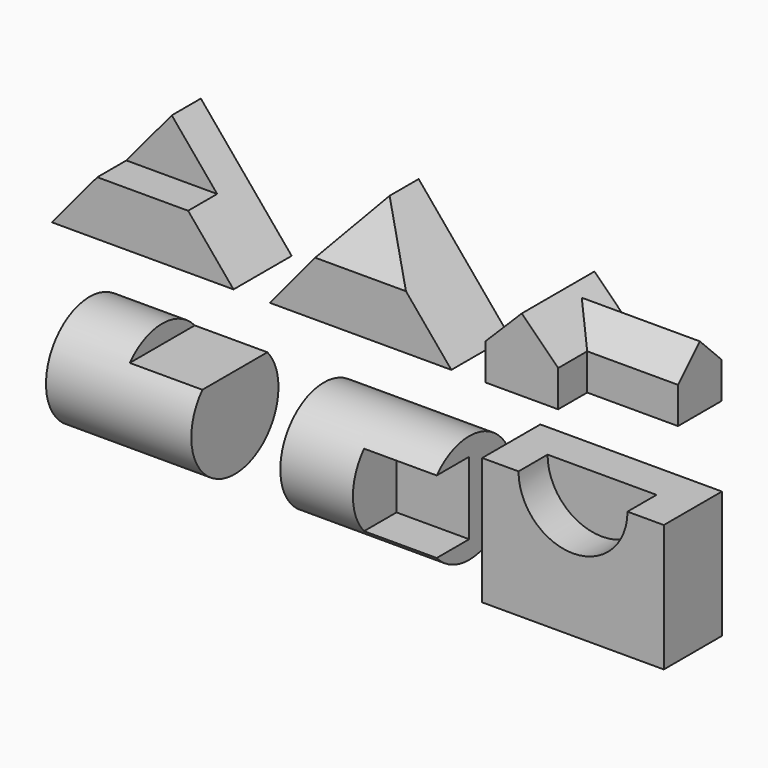
from build123d import *

# Parameters (mm, degrees)
F1_DEPTH  = 101.6
F3_DEPTH  = 50.8
F5_DEPTH  = 101.6
F9_DEPTH  = 63.5
F11_DEPTH = 127
F15_R     = 76.2
F16_DEPTH = 203.2
F18_DEPTH = 101.6
F20_R     = 76.2
F21_DEPTH = 203.2
F23_DEPTH = 101.6
F25_DEPTH = 101.6
F27_DEPTH = 50.8


with BuildPart() as f1:
    # F0 (on Front) → F1 (new body)
    with BuildSketch(Plane.XZ):
        Polygon((127, 152.4), (0, 0), (254, 0), align=None)
    extrude(amount=-F1_DEPTH)

    # F2 (on face) → F3 (cut)
    with BuildSketch(Plane.XZ):
        Polygon((63.5, 76.2), (127, 76.2), (190.5, 76.2), (127, 152.4), align=None)
    extrude(amount=-F3_DEPTH, mode=Mode.SUBTRACT)


with BuildPart() as f5:
    # F4 (on Front) → F5 (new body)
    with BuildSketch(Plane.XZ):
        Polygon((431.6333237171, 152.4), (304.6333237171, 0), (558.6333237171, 0), align=None)
    extrude(amount=-F5_DEPTH)

    # F8 (on 3pt) → F9 (cut, symmetric)
    with BuildSketch(Plane.YZ.offset(431.6333237171)):
        Polygon((50.8, 152.4), (0, 152.4), (0, 76.2), align=None)
    extrude(amount=F9_DEPTH, both=True, mode=Mode.SUBTRACT)


with BuildPart() as f11:
    # F10 (on Front) → F11 (new body)
    with BuildSketch(Plane.XZ):
        Polygon((606.3837154388, 50.8), (606.3837154388, 0), (657.1837154388, 0), (707.9837154388, 0), (707.9837154388, 50.8), (657.1837154388, 101.6), align=None)
    extrude(amount=-F11_DEPTH)

    # F13 (on offset) → F14 (join, up to the next surface of F11)
    with BuildSketch(Plane.YZ.offset(834.9837154388)):
        Polygon((88.9, 88.9), (50.8, 50.8), (50.8, 0), (127, 0), (127, 50.8), align=None)
    extrude(until=Until.NEXT, dir=(-1, 0, 0))


with BuildPart() as f16:
    # F15 (on Right) → F16 (new body)
    with BuildSketch(Plane.YZ):
        with Locations((65.8603087068, -194.5504695177)):
            Circle(F15_R)
    extrude(amount=F16_DEPTH)

    # F17 (on face) → F18 (cut)
    with BuildSketch(Plane.YZ.offset(203.2)):
        with BuildLine():
            Line((9.0641820783, -143.7504695177), (65.8603087068, -143.7504695177))
            Line((65.8603087068, -143.7504695177), (122.6564353353, -143.7504695177))
            ThreePointArc((122.6564353353, -143.7504695177), (65.8603087068, -118.3504695177), (9.0641820783, -143.7504695177))
        make_face()
    extrude(amount=-F18_DEPTH, mode=Mode.SUBTRACT)


with BuildPart() as f21:
    # F20 (on offset) → F21 (new body)
    with BuildSketch(Plane.YZ.offset(327.66)):
        with Locations((65.8921543072, -193.5252969361)):
            Circle(F20_R)
    extrude(amount=F21_DEPTH)

    # F22 (on face) → F23 (cut)
    with BuildSketch(Plane.YZ.offset(530.86)):
        with BuildLine():
            Line((65.8921543072, -244.3252969361), (65.8921543072, -142.7252969361))
            Line((65.8921543072, -142.7252969361), (9.0960276787, -142.7252969361))
            ThreePointArc((9.0960276787, -142.7252969361), (-10.3078456928, -193.5252969361), (9.0960276787, -244.3252969361))
            Line((9.0960276787, -244.3252969361), (65.8921543072, -244.3252969361))
        make_face()
    extrude(amount=-F23_DEPTH, mode=Mode.SUBTRACT)


with BuildPart() as f25:
    # F24 (on Front) → F25 (new body)
    with BuildSketch(Plane.XZ):
        Polygon((601.7486453056, -94.4223997116), (601.7486453056, -272.2223997116), (855.7486453056, -272.2223997116), (855.7486453056, -94.4223997116), (804.9486453056, -94.4223997116), (652.5486453056, -94.4223997116), align=None)
    extrude(amount=-F25_DEPTH)

    # F26 (on face) → F27 (cut)
    with BuildSketch(Plane.XZ):
        with BuildLine():
            Line((804.9486453056, -94.4223997116), (652.5486453056, -94.4223997116))
            ThreePointArc((652.5486453056, -94.4223997116), (728.7486453056, -170.6223997116), (804.9486453056, -94.4223997116))
        make_face()
    extrude(amount=-F27_DEPTH, mode=Mode.SUBTRACT)


solid = Compound([f1.part, f5.part, f11.part, f16.part, f21.part, f25.part])
